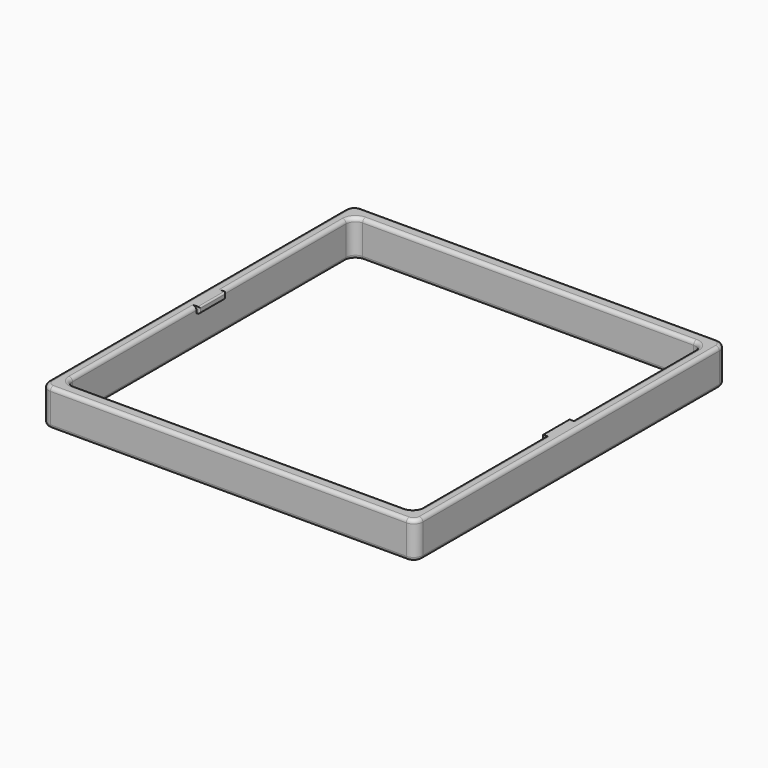
from build123d import *

# Parameters (mm, degrees)
F0_W     = 129.54
F0_H     = 134.62
F0_W_2   = 120.904
F0_H_2   = 124.714
F1_DEPTH = 12.7
F2_R     = 3.175
F4_W     = 11.43
F4_H     = 2.159
F5_DEPTH = 1.016
F3_W     = 11.43
F3_H     = 2.159
F6_DEPTH = 1.016
F7_R     = 1.27
F8_R     = 0.508
F10_R    = 1.27


with BuildPart() as f1:
    # F0 (on Top) → F1 (new body)
    with BuildSketch(Plane.XY):
        Rectangle(F0_W, F0_H)
        Rectangle(F0_W_2, F0_H_2, mode=Mode.SUBTRACT)
    extrude(amount=F1_DEPTH)

    # F2
    f2_edges = [f1.edges().sort_by_distance(p)[0] for p in [
        (-60.452, 62.357, 6.35),
        (-60.452, -62.357, 6.35),
        (60.452, 62.357, 6.35),
        (60.452, -62.357, 6.35),
        (-64.77, 67.31, 6.35),
        (64.77, 67.31, 6.35),
        (-64.77, -67.31, 6.35),
        (64.77, -67.31, 6.35),
    ]]
    fillet(f2_edges, radius=F2_R)

    # F4 (on face) → F5 (join)
    with BuildSketch(Plane(origin=(60.452, 0, 0), x_dir=(0, -1, 0), z_dir=(-1, 0, 0))):
        with Locations((0.127, 11.6205)):
            Rectangle(F4_W, F4_H)
    extrude(amount=F5_DEPTH)

    # F3 (on face) → F6 (join)
    with BuildSketch(Plane.YZ.offset(-60.452)):
        with Locations((0.127, 11.6205)):
            Rectangle(F3_W, F3_H)
    extrude(amount=F6_DEPTH)

    # F7
    f7_edges = [f1.edges().sort_by_distance(p)[0] for p in [
        (0, -62.357, 12.7),
        (0, 62.357, 0),
        (-64.77, 0, 0),
        (-60.452, 32.512, 12.7),
    ]]
    fillet(f7_edges, radius=F7_R)

    # F8
    f8_edges = [f1.edges().sort_by_distance(p)[0] for p in [
        (-59.436, 5.842, 11.6205),
        (-59.436, -5.588, 11.6205),
        (-59.436, 0.127, 10.541),
        (-59.436, 0.127, 12.7),
        (59.436, 5.588, 11.6205),
        (59.436, -5.842, 11.6205),
        (59.436, -0.127, 12.7),
        (59.436, -0.127, 10.541),
    ]]
    fillet(f8_edges, radius=F8_R)

    # F10
    f10_edges = [f1.edges().sort_by_distance(p)[0] for p in [
        (0, 67.31, 12.7),
        (-63.840064, 66.380064, 12.7),
        (-64.77, 0, 12.7),
        (-63.840064, -66.380064, 12.7),
        (0, -67.31, 12.7),
        (63.840064, -66.380064, 12.7),
        (64.77, 0, 12.7),
        (63.840064, 66.380064, 12.7),
    ]]
    fillet(f10_edges, radius=F10_R)


solid = f1.part
